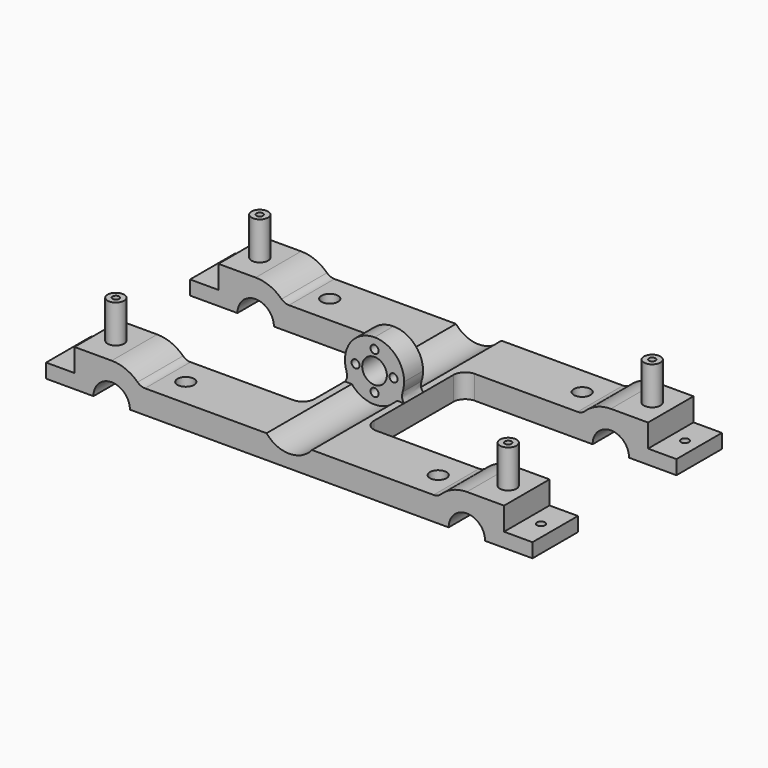
from build123d import *

# Parameters (mm, degrees)
F0_R      = 3.5
F1_DEPTH  = 10
F0_W      = 31.4
F0_H      = 24
F2_DEPTH  = 15.7
F3_DEPTH  = 30.5
F6_DEPTH  = 100
F7_R      = 1.7
F7_R_2    = 5.2
F8_DEPTH  = 60
F9_DEPTH  = 100
F10_DEPTH = 100
F11_DEPTH = 10
F12_R     = 5
F0_W_2    = 12
F0_R_2    = 1.7
F13_DEPTH = 6
F14_DEPTH = 6
F15_R     = 3.5
F15_R_2   = 1.4
F16_DEPTH = 16


# Not quite as in the source:
# - a feature names something its author has since deleted; it is built from what else it names


with BuildPart() as f1:
    # F0 (on Top) → F1 (new body)
    with BuildSketch(Plane.XY):
        Polygon((59.3, 50), (0, 50), (-59.3, 50), (-59.3, 26), (-12.5, 26), (-12.5, 5), (12.5, 5), (12.5, 26), (59.3, 26), align=None)
        with Locations((-53.3, 38)):
            Circle(F0_R, mode=Mode.SUBTRACT)
        with Locations((53.3, 38)):
            Circle(F0_R, mode=Mode.SUBTRACT)
    extrude(amount=F1_DEPTH)

    # F0 (on Top) → F2 (join)
    with BuildSketch(Plane.XY):
        with Locations((-75, 38)):
            Rectangle(F0_W, F0_H)
        with Locations((75, 38)):
            Rectangle(F0_W, F0_H)
    extrude(amount=F2_DEPTH)



with BuildPart() as f1b:
    # F0 (on Top) → F1, piece 2 (new body)
    with BuildSketch(Plane.XY):
        Polygon((12.5, -5), (-12.5, -5), (-12.5, -26), (-59.3, -26), (-59.3, -50), (0, -50), (59.3, -50), (59.3, -26), (12.5, -26), align=None)
        with Locations((-53.3, -38)):
            Circle(F0_R, mode=Mode.SUBTRACT)
        with Locations((53.3, -38)):
            Circle(F0_R, mode=Mode.SUBTRACT)
    extrude(amount=F1_DEPTH)

    # F0 (on Top) → F2, piece 2 (join)
    with BuildSketch(Plane.XY):
        with Locations((-75, -38)):
            Rectangle(F0_W, F0_H)
        with Locations((75, -38)):
            Rectangle(F0_W, F0_H)
    extrude(amount=F2_DEPTH)


with BuildPart() as f1_1:
    add(f1.part)

    add(f1b.part)  # F3 merges F1b
    # F0 (on Top) → F3 (join)
    with BuildSketch(Plane.XY):
        Polygon((12.5, 5), (-12.5, 5), (-12.5, 0), (-12.5, -5), (12.5, -5), (12.5, 0), align=None)
    extrude(amount=F3_DEPTH)

    # F4: union 

    # F5 (on face) → F6 (cut)
    with BuildSketch(Plane.XZ.offset(50)):
        with BuildLine():
            Line((59.3, 15.7), (59.3, 10))
            Line((59.3, 10), (60.936808709, 10))
            ThreePointArc((60.936808709, 10), (62.6266035374, 10.3294327596), (64.0689074703, 11.2694816254))
            ThreePointArc((64.0689074703, 11.2694816254), (69.1025794418, 14.5502725321), (75, 15.7))
            Line((75, 15.7), (59.3, 15.7))
        make_face()
        with BuildLine():
            ThreePointArc((82.7, 0), (75, 7.7), (67.3, 0))
            Line((67.3, 0), (82.7, 0))
        make_face()
        with BuildLine():
            ThreePointArc((-75, 15.7), (-69.1025794418, 14.5502725321), (-64.0689074703, 11.2694816254))
            ThreePointArc((-64.0689074703, 11.2694816254), (-62.6266035374, 10.3294327596), (-60.936808709, 10))
            Line((-60.936808709, 10), (-59.3, 10))
            Line((-59.3, 10), (-59.3, 15.7))
            Line((-59.3, 15.7), (-75, 15.7))
        make_face()
        with BuildLine():
            ThreePointArc((-67.3, 0), (-75, 7.7), (-82.7, 0))
            Line((-82.7, 0), (-67.3, 0))
        make_face()
    extrude(amount=-F6_DEPTH, mode=Mode.SUBTRACT)

    # F7 (on face) → F8 (cut, symmetric)
    with BuildSketch(Plane.XZ.offset(5)):
        with BuildLine():
            Line((-12.5, 30.5), (-12.5, 18))
            ThreePointArc((-12.5, 18), (-8.8388347819, 26.8388347478), (-4.83e-08, 30.5))
            Line((-4.83e-08, 30.5), (-12.5, 30.5))
        make_face()
        with BuildLine():
            Line((12.5, 30.5), (-4.83e-08, 30.5))
            ThreePointArc((-4.83e-08, 30.5), (8.8388347478, 26.8388347819), (12.5, 18))
            Line((12.5, 18), (12.5, 30.5))
        make_face()
        with BuildLine():
            add(Edge.make_bspline(
                [(-11.8176156762, 13.9264315731), (-11.6747882381, 13.1368398711), (-11.3919431578, 11.6323543495), (-12.1435697242, 10.5264146596), (-12.5, 10)],
                knots=[0, 0, 0, 0, 0.5238869887, 1, 1, 1, 1], degree=3))
            ThreePointArc((-11.8176156762, 13.9264315731), (-12.3282236343, 15.9348360783), (-12.5, 18))
            Line((-12.5, 18), (-12.5, 10))
        make_face()
        with BuildLine():
            Line((12.5, 10), (12.5, 18))
            ThreePointArc((12.5, 18), (12.3282236343, 15.9348360783), (11.8176156762, 13.9264315731))
            add(Edge.make_bspline(
                [(11.8176156762, 13.9264315731), (11.6747882381, 13.1368398711), (11.3919431578, 11.6323543495), (12.1435697242, 10.5264146596), (12.5, 10)],
                knots=[0, 0, 0, 0, 0.5238869887, 1, 1, 1, 1], degree=3))
        make_face()
        with Locations((-8, 18)):
            Circle(F7_R)
        with Locations((0, 26)):
            Circle(F7_R)
        with Locations((8, 18)):
            Circle(F7_R)
        with BuildLine():
            ThreePointArc((1.7, 10), (0, 11.7), (-1.7, 10))
            Line((-1.7, 10), (1.7, 10))
        make_face()
        with BuildLine():
            Line((1.7, 10), (-1.7, 10))
            ThreePointArc((-1.7, 10), (0, 8.3), (1.7, 10))
        make_face()
        with Locations((0, 18)):
            Circle(F7_R_2)
    extrude(amount=F8_DEPTH, both=True, mode=Mode.SUBTRACT)

    # F7 (on face) → F9 (cut)
    with BuildSketch(Plane.XZ.offset(5)):
        with BuildLine():
            Line((-1.7, 10), (-9.6046863561, 10))
            ThreePointArc((-9.6046863561, 10), (0, 5.5), (9.6046863561, 10))
            Line((9.6046863561, 10), (1.7, 10))
            ThreePointArc((1.7, 10), (0, 8.3), (-1.7, 10))
        make_face()
    extrude(amount=F9_DEPTH, mode=Mode.SUBTRACT)

    # F7 (on face) → F10 (cut)
    with BuildSketch(Plane.XZ.offset(5)):
        with BuildLine():
            Line((-1.7, 10), (-9.6046863561, 10))
            ThreePointArc((-9.6046863561, 10), (0, 5.5), (9.6046863561, 10))
            Line((9.6046863561, 10), (1.7, 10))
            ThreePointArc((1.7, 10), (0, 8.3), (-1.7, 10))
        make_face()
    extrude(amount=-F10_DEPTH, mode=Mode.SUBTRACT)

    # F7 (on face) → F11 (join)
    with BuildSketch(Plane.XZ.offset(5)):
        with BuildLine():
            Line((-1.7, 10), (-9.6046863561, 10))
            ThreePointArc((-9.6046863561, 10), (0, 5.5), (9.6046863561, 10))
            Line((9.6046863561, 10), (1.7, 10))
            ThreePointArc((1.7, 10), (0, 8.3), (-1.7, 10))
        make_face()
    extrude(amount=-F11_DEPTH)

    # F12
    f12_edges = [f1_1.edges().sort_by_distance(p)[0] for p in [
        (-12.5, 26, 5),
        (12.5, 26, 5),
        (-12.5, -26, 5),
        (12.5, -26, 5),
    ]]
    fillet(f12_edges, radius=F12_R)

    # F0 (on Top) → F13 (join)
    with BuildSketch(Plane.XY):
        with Locations((-96.7, 38)):
            Rectangle(F0_W_2, F0_H)
        with Locations((-96.7, 38)):
            Circle(F0_R_2, mode=Mode.SUBTRACT)
        with Locations((-96.7, -38)):
            Rectangle(F0_W_2, F0_H)
        with Locations((-96.7, -38)):
            Circle(F0_R_2, mode=Mode.SUBTRACT)
        with Locations((96.7, -38)):
            Rectangle(F0_W_2, F0_H)
        with Locations((96.7, -38)):
            Circle(F0_R_2, mode=Mode.SUBTRACT)
        with Locations((96.7, 38)):
            Rectangle(F0_W_2, F0_H)
        with Locations((96.7, 38)):
            Circle(F0_R_2, mode=Mode.SUBTRACT)
    extrude(amount=F13_DEPTH)

    # F0 (on Top) → F14 (join)
    with BuildSketch(Plane.XY):
        with Locations((-53.3, 38)):
            Circle(F0_R)
        with Locations((-53.3, 38)):
            Circle(F0_R_2, mode=Mode.SUBTRACT)
        with Locations((53.3, 38)):
            Circle(F0_R)
        with Locations((53.3, 38)):
            Circle(F0_R_2, mode=Mode.SUBTRACT)
        with Locations((-53.3, -38)):
            Circle(F0_R)
        with Locations((-53.3, -38)):
            Circle(F0_R_2, mode=Mode.SUBTRACT)
        with Locations((53.3, -38)):
            Circle(F0_R)
        with Locations((53.3, -38)):
            Circle(F0_R_2, mode=Mode.SUBTRACT)
    extrude(amount=F14_DEPTH)

    # F15 (on face) → F16 (join)
    with BuildSketch(Plane.XY.offset(15.7)):
        with Locations((-82.85, 38)):
            Circle(F15_R)
        with Locations((-82.85, 38)):
            Circle(F15_R_2, mode=Mode.SUBTRACT)
        with Locations((82.85, 38)):
            Circle(F15_R)
        with Locations((82.85, 38)):
            Circle(F15_R_2, mode=Mode.SUBTRACT)
        with Locations((82.85, -38)):
            Circle(F15_R)
        with Locations((82.85, -38)):
            Circle(F15_R_2, mode=Mode.SUBTRACT)
        with Locations((-82.85, -38)):
            Circle(F15_R)
        with Locations((-82.85, -38)):
            Circle(F15_R_2, mode=Mode.SUBTRACT)
    extrude(amount=F16_DEPTH)


solid = f1_1.part
